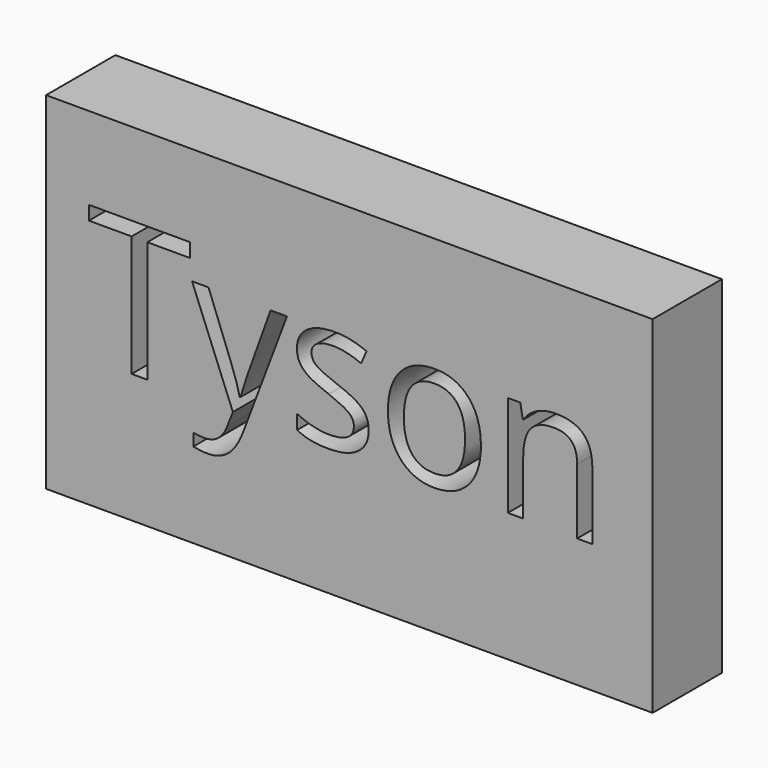
from build123d import *

# Parameters (mm, degrees)
F0_W         = 177.8
F0_H         = 101.6
F1_DEPTH     = 25.4
F3_TEXT_SIZE = 55.4335678721
F4_DEPTH     = 19.05


# Not quite as in the source:
# - Text() gives the source's letters only with a copy of the font that has no kerning and outlines rounded to 1/6400 em; it was checked with that copy


with BuildPart() as f1:
    # F0 (on Front) → F1 (new body)
    with BuildSketch(Plane.XZ):
        with Locations((-29.5769619516, -2.7991831303)):
            Rectangle(F0_W, F0_H)
    extrude(amount=F1_DEPTH)

    # F3 (on face) → F4 (cut)
    with BuildSketch(Plane.XZ.offset(25.4)):
        with Locations((-106.4124777913, -15.7923847437)):
            Text('Tyson', F3_TEXT_SIZE, font='Open Sans', text_align=(TextAlign.LEFT, TextAlign.BOTTOM))
    extrude(amount=-F4_DEPTH, mode=Mode.SUBTRACT)


solid = f1.part
